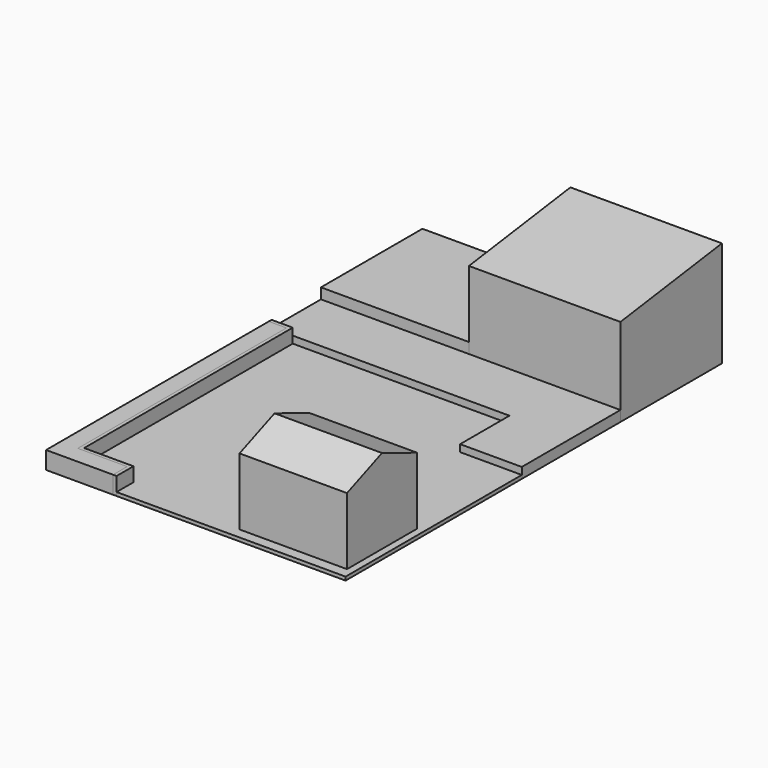
from build123d import *

# Parameters (mm, degrees)
F0_W        = 3050
F0_H        = 2483
F0_W_2      = 500
F0_H_2      = 100
F0_W_3      = 1750
F0_H_3      = 1750
F0_W_4      = 4200
F0_H_4      = 3600
F1_DEPTH    = 100
F2_DEPTH    = 500
F3_DEPTH    = 300
F4_DEPTH    = 600
F5_DEPTH    = 2500
F6_T1_DEPTH = 9532.7840978253
F0_W_5      = 100
F7_DEPTH    = 500
F0_W_6      = 4300
F8_DEPTH    = 3000
F9_SIZE2    = 499.99999
F9_SIZE     = 3599.99999


# Not quite as in the source:
# - a fillet or chamfer that OpenCascade refuses, or shapes differently, is made with other operations: its cross-section is extruded or revolved along the edge and cut away or added
# - a fillet or chamfer is up to 0.001 mm smaller than in the source, because OpenCascade refuses the exact size


with BuildPart() as f1:
    # F0 (on Top) → F1 (new body)
    with BuildSketch(Plane.XY):
        Polygon((2500, -1750), (2500, 0), (-3650, 0), (-3650, -100), (-3650, -7400), (-2250, -7400), (-2250, -8000), (4250, -8000), (4250, -1750), align=None)
        with Locations((2525, -6458.5)):
            Rectangle(F0_W, F0_H, mode=Mode.SUBTRACT)
        with Locations((2525, -6458.5)):
            Rectangle(F0_W, F0_H)
        with Locations((-4000, -50)):
            Rectangle(F0_W_2, F0_H_2)
        with Locations((3375, -875)):
            Rectangle(F0_W_3, F0_H_3)
        Polygon((2500, 0), (4250, 0), (4250, 1750), (-50, 1750), (-4250, 1750), (-4250, 0), (-3750, 0), (-3650, 0), align=None)
        with Locations((-2150, 3550)):
            Rectangle(F0_W_4, F0_H_4)
    extrude(amount=F1_DEPTH)


with BuildPart() as f2:
    # F0 (on Top) → F2 (new body)
    with BuildSketch(Plane.XY):
        Polygon((-3750, -7500), (-3750, -100), (-4250, -100), (-4250, -8000), (-2350, -8000), (-2350, -7500), align=None)
    extrude(amount=F2_DEPTH)


with BuildPart() as f3:
    # F0 (on Top) → F3 (new body)
    with BuildSketch(Plane.XY):
        Polygon((2500, 0), (4250, 0), (4250, 1750), (-50, 1750), (-4250, 1750), (-4250, 0), (-3750, 0), (-3650, 0), align=None)
        with Locations((3375, -875)):
            Rectangle(F0_W_3, F0_H_3)
    extrude(amount=F3_DEPTH)


with BuildPart() as f4:
    # F0 (on Top) → F4 (new body)
    with BuildSketch(Plane.XY):
        with Locations((-2150, 3550)):
            Rectangle(F0_W_4, F0_H_4)
    extrude(amount=F4_DEPTH)


with BuildPart() as f5:
    # F0 (on Top) → F5 (new body)
    with BuildSketch(Plane.XY):
        with Locations((2525, -6458.5)):
            Rectangle(F0_W, F0_H)
    extrude(amount=F5_DEPTH)

    # F6: chamfer of 500 x 1250 on 2 edges, made by hand

    # F6_s2 → F6_t1 (cut)
    with BuildSketch(Plane.YZ.offset(-2241.3920489126)):
        Polygon((-7700, 2000), (-6450, 2500), (-7700, 2500), align=None)
        Polygon((-5217, 2000), (-6467, 2500), (-5217, 2500), align=None)
    extrude(amount=F6_T1_DEPTH, mode=Mode.SUBTRACT)


with BuildPart() as f7:
    # F0 (on Top) → F7 (new body, through all)
    with BuildSketch(Plane.XY):
        with Locations((-3700, -50)):
            Rectangle(F0_W_5, F0_H_2)
        Polygon((-3650, -7400), (-3650, -100), (-3750, -100), (-3750, -7500), (-2350, -7500), (-2350, -8000), (-2250, -8000), (-2250, -7400), align=None)
        with Locations((-4000, -50)):
            Rectangle(F0_W_2, F0_H_2)
    extrude(amount=F7_DEPTH)


with BuildPart() as f8:
    # F0 (on Top) → F8 (new body)
    with BuildSketch(Plane.XY):
        with Locations((2100, 3550)):
            Rectangle(F0_W_6, F0_H_4)
    extrude(amount=F8_DEPTH)

    # F9 (size 3600 and 500 in the source; OpenCascade refuses exactly that, so slightly less here)
    f9_edges = [f8.edges().sort_by_distance(p)[0] for p in [
        (2100, 1750, 3000),
    ]]
    f9_side = f8.faces().sort_by_distance((2100, 3550, 3000))[0]
    chamfer(f9_edges, length=F9_SIZE, length2=F9_SIZE2, reference=f9_side)


solid = Compound([f1.part, f2.part, f3.part, f4.part, f5.part, f7.part, f8.part])
